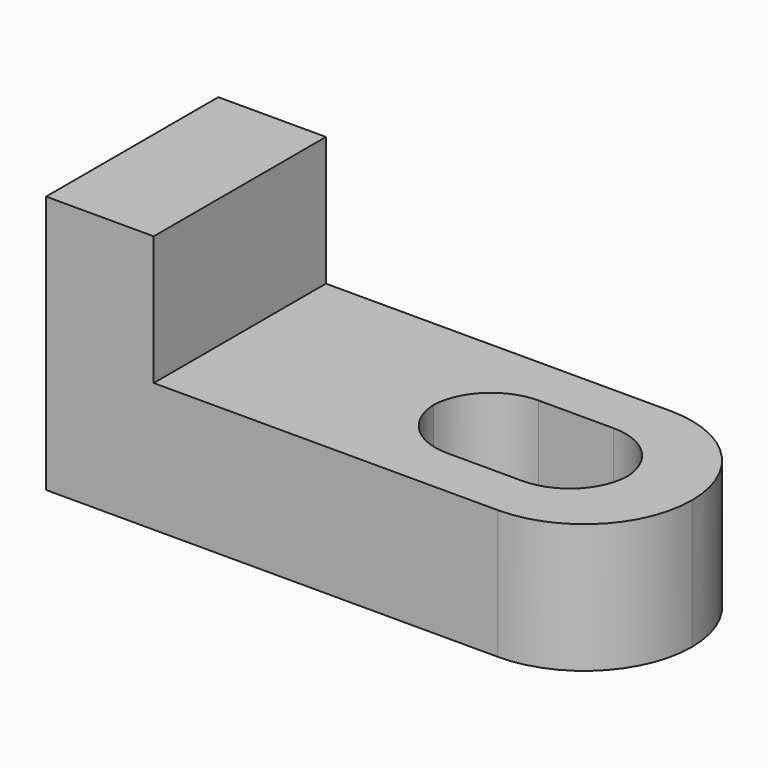
from build123d import *

# Parameters (mm, degrees)
F0_W        = 21
F0_H        = 10
F0_W_2      = 9
F0_H_2      = 5.3
F0_W_3      = 5
F1_DEPTH    = 6
F2_DEPTH    = 12
F3_T1_DEPTH = 6
F4_R        = 4.99999


# Not quite as in the source:
# - a fillet or chamfer that OpenCascade refuses, or shapes differently, is made with other operations: its cross-section is extruded or revolved along the edge and cut away or added
# - a fillet or chamfer is up to 0.001 mm smaller than in the source, because OpenCascade refuses the exact size


with BuildPart() as f1:
    # F0 (on Top) → F1 (new body)
    with BuildSketch(Plane.XY):
        with Locations((-10.5, 5)):
            Rectangle(F0_W, F0_H)
        with Locations((-7.5, 5)):
            Rectangle(F0_W_2, F0_H_2, mode=Mode.SUBTRACT)
        with Locations((-23.5, 5)):
            Rectangle(F0_W_3, F0_H)
    extrude(amount=F1_DEPTH)

    # F0 (on Top) → F2 (join)
    with BuildSketch(Plane.XY):
        with Locations((-23.5, 5)):
            Rectangle(F0_W_3, F0_H)
    extrude(amount=F2_DEPTH)

    # F3: fillet of radius 2.75 on 4 edges, made by hand

    # F3_s2 → F3_t1 (join)
    with BuildSketch(Plane.XY):
        with BuildLine():
            ThreePointArc((-9.25, 7.65), (-11.1945436483, 6.8445436483), (-12, 4.9))
            Line((-12, 4.9), (-12, 7.65))
            Line((-12, 7.65), (-9.25, 7.65))
        make_face()
        with BuildLine():
            ThreePointArc((-12, 5.1), (-11.1945436483, 3.1554563517), (-9.25, 2.35))
            Line((-9.25, 2.35), (-12, 2.35))
            Line((-12, 2.35), (-12, 5.1))
        make_face()
        with BuildLine():
            ThreePointArc((-5.75, 7.65), (-3.8054563517, 6.8445436483), (-3, 4.9))
            Line((-3, 4.9), (-3, 7.65))
            Line((-3, 7.65), (-5.75, 7.65))
        make_face()
        with BuildLine():
            ThreePointArc((-3, 5.1), (-3.8054563517, 3.1554563517), (-5.75, 2.35))
            Line((-5.75, 2.35), (-3, 2.35))
            Line((-3, 2.35), (-3, 5.1))
        make_face()
    extrude(amount=F3_T1_DEPTH)

    # F4 (radius 5 in the source; OpenCascade refuses exactly that, so slightly less here)
    f4_edges = [f1.edges().sort_by_distance(p)[0] for p in [
        (0, 0, 3),
        (0, 10, 3),
    ]]
    fillet(f4_edges, radius=F4_R)


solid = f1.part
